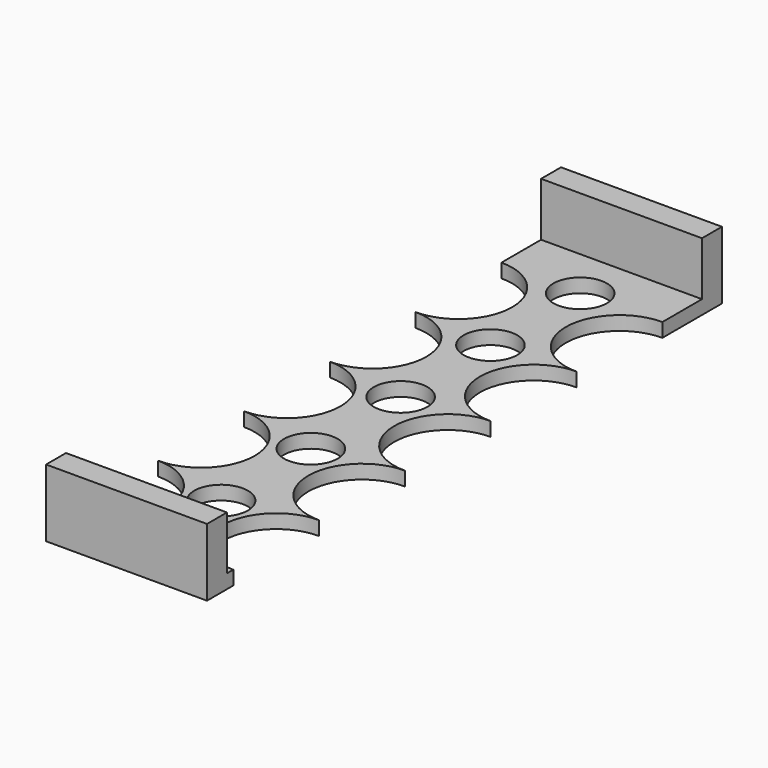
from build123d import *

# Parameters (mm, degrees)
F0_W     = 38.1
F0_H     = 152.4
F0_R     = 6.35
F1_DEPTH = 3.302
F2_W     = 38.1
F2_H     = 5.8965822577
F3_DEPTH = 12.7
F5_DEPTH = 25.4


with BuildPart() as f1:
    # F0 (on Top) → F1 (new body)
    with BuildSketch(Plane.XY):
        Rectangle(F0_W, F0_H)
        with Locations((0, -48.2141543601)):
            Circle(F0_R, mode=Mode.SUBTRACT)
        with Locations((0, -21.6441029067)):
            Circle(F0_R, mode=Mode.SUBTRACT)
        with Locations((0, 4.9259485466)):
            Circle(F0_R, mode=Mode.SUBTRACT)
        with Locations((0, 31.496)):
            Circle(F0_R, mode=Mode.SUBTRACT)
        with Locations((0, 58.0660514534)):
            Circle(F0_R, mode=Mode.SUBTRACT)
    extrude(amount=F1_DEPTH)

    # F2 (on face) → F3 (join)
    with BuildSketch(Plane.XY.offset(3.302)):
        with Locations((0, 73.2517088711)):
            Rectangle(F2_W, F2_H)
        with Locations((0, -73.2517088711)):
            Rectangle(F2_W, F2_H)
    extrude(amount=F3_DEPTH)

    # F4 (on face) → F5 (cut)
    with BuildSketch(Plane.XY.offset(3.302)):
        with BuildLine():
            ThreePointArc((-19.05, 33.1740033209), (-10.0697438789, 36.8937471999), (-6.35, 45.8740033209))
            ThreePointArc((-6.35, 45.8740033209), (-10.0697438789, 54.854259442), (-19.05, 58.5740033209))
            Line((-19.05, 58.5740033209), (-19.05, 33.1740033209))
        make_face()
        with BuildLine():
            ThreePointArc((-6.35, 20.4740033209), (-10.0697438789, 29.454259442), (-19.05, 33.1740033209))
            Line((-19.05, 33.1740033209), (-19.05, 7.7740033209))
            ThreePointArc((-19.05, 7.7740033209), (-10.0697438789, 11.4937471999), (-6.35, 20.4740033209))
        make_face()
        with BuildLine():
            ThreePointArc((-6.35, -4.9259966791), (-10.0697438789, 4.054259442), (-19.05, 7.7740033209))
            Line((-19.05, 7.7740033209), (-19.05, -17.6259966791))
            ThreePointArc((-19.05, -17.6259966791), (-10.0697438789, -13.9062528001), (-6.35, -4.9259966791))
        make_face()
        with BuildLine():
            ThreePointArc((-6.35, -30.3259966791), (-10.0697438789, -21.345740558), (-19.05, -17.6259966791))
            Line((-19.05, -17.6259966791), (-19.05, -43.0259966791))
            ThreePointArc((-19.05, -43.0259966791), (-10.0697438789, -39.3062528001), (-6.35, -30.3259966791))
        make_face()
        with BuildLine():
            Line((19.05, 33.1740033209), (19.05, 58.5740033209))
            ThreePointArc((19.05, 58.5740033209), (6.35, 45.8740033209), (19.05, 33.1740033209))
        make_face()
        with BuildLine():
            ThreePointArc((-6.35, -55.7259966791), (-10.0697438789, -46.745740558), (-19.05, -43.0259966791))
            Line((-19.05, -43.0259966791), (-19.05, -68.4259966791))
            ThreePointArc((-19.05, -68.4259966791), (-10.0697438789, -64.7062528001), (-6.35, -55.7259966791))
        make_face()
        with BuildLine():
            Line((19.05, 7.7740033209), (19.05, 33.1740033209))
            ThreePointArc((19.05, 33.1740033209), (6.35, 20.4740033209), (19.05, 7.7740033209))
        make_face()
        with BuildLine():
            Line((19.05, -17.6259966791), (19.05, 7.7740033209))
            ThreePointArc((19.05, 7.7740033209), (6.35, -4.9259966791), (19.05, -17.6259966791))
        make_face()
        with BuildLine():
            Line((19.05, -43.0259966791), (19.05, -17.6259966791))
            ThreePointArc((19.05, -17.6259966791), (6.35, -30.3259966791), (19.05, -43.0259966791))
        make_face()
        with BuildLine():
            Line((19.05, -68.4259966791), (19.05, -43.0259966791))
            ThreePointArc((19.05, -43.0259966791), (6.35, -55.7259966791), (19.05, -68.4259966791))
        make_face()
    extrude(amount=-F5_DEPTH, mode=Mode.SUBTRACT)


solid = f1.part
